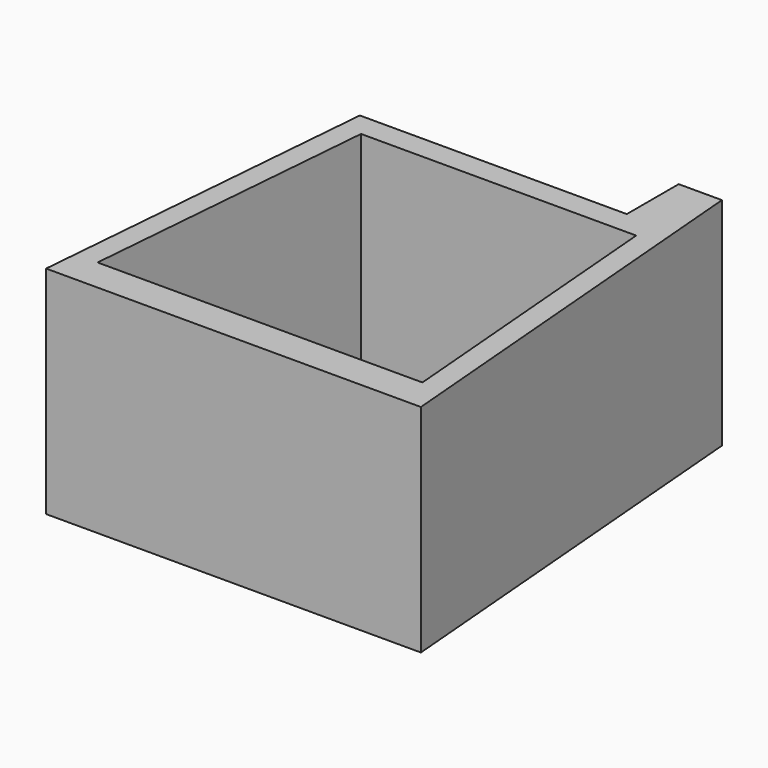
from build123d import *

# Parameters (mm, degrees)
F1_DEPTH = 20


# Not quite as in the source:
# - a feature names something its author has since deleted; it is built from what else it names


with BuildPart() as f1:
    # F0 (on Top) → F1 (new body)
    with BuildSketch(Plane.XY):
        Polygon((0, 15.9851339135), (-10.1, 15.9851339135), (-14.6001070377, 15.9851339135), (-17.3394622729, -16.880093272), (0, -16.880093272), (17.3394622729, -16.880093272), (14.1, 21.9851339135), (10.1, 21.9851339135), (10.1, 15.9851339135), align=None)
        Polygon((11.9072113089, -13.8146081649), (-11.9072113089, -13.8146081649), (-15.0287533179, -13.8146081649), (-12.7284283152, 13.7833838166), (-9.6068863062, 13.7833838166), (0, 13.7833838166), (9.6068863062, 13.7833838166), (12.7284283152, 13.7833838166), (15.0287533179, -13.8146081649), align=None, mode=Mode.SUBTRACT)
    extrude(amount=F1_DEPTH)


solid = f1.part
